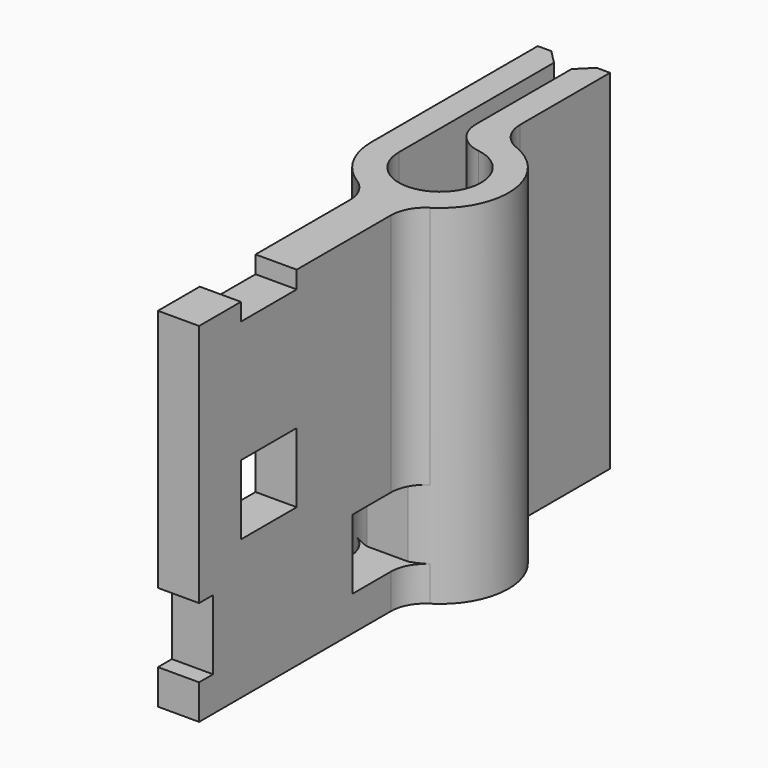
from build123d import *

# Parameters (mm, degrees)
F1_DEPTH = 25.4
F2_SIZE  = 1.016
F3_W     = 3
F3_H     = 19.05
F4_DEPTH = 25.4
F5_W     = 5.08
F5_H     = 5.08
F5_W_2   = 1.27
F5_H_2   = 1.27
F6_DEPTH = 6.501
F7_R     = 2.5


with BuildPart() as f1:
    # F0 (on Top) → F1 (new body)
    with BuildSketch(Plane.XY):
        with BuildLine():
            Line((0.635, 15.1509385957), (0.635, 2.4509385957))
            ThreePointArc((0.635, 2.4509385957), (5.0286441204, -1.3802173742), (-0.635, 0))
            Line((-0.635, 0), (-0.635, 15.1509385957))
            Line((-0.635, 15.1509385957), (-2.635, 15.1509385957))
            Line((-2.635, 15.1509385957), (-2.635, 0))
            ThreePointArc((-2.635, 0), (5.8037497728, -3.6297382826), (2.635, 4.9927046778))
            Line((2.635, 4.9927046778), (2.635, 15.1509385957))
            Line((2.635, 15.1509385957), (0.635, 15.1509385957))
        make_face()
    extrude(amount=F1_DEPTH)

    # F2
    f2_edges = [f1.edges().sort_by_distance(p)[0] for p in [
        (-0.635, 15.150939, 12.7),
        (0.635, 15.150939, 12.7),
    ]]
    chamfer(f2_edges, length=F2_SIZE)

    # F3 (on Top) → F4 (join, through all)
    with BuildSketch(Plane.XY):
        with Locations((2.365, -14.2946960071)):
            Rectangle(F3_W, F3_H)
    extrude(amount=F4_DEPTH)

    # F5 (on face) → F6 (cut, through all)
    with BuildSketch(Plane.YZ.offset(3.865)):
        with Locations((-7.3096960071, 5.08)):
            Rectangle(F5_W, F5_H)
        with Locations((-17.4696960071, 12.7)):
            Rectangle(F5_W, F5_H)
        with Locations((-23.1846960071, 5.08)):
            Rectangle(F5_W_2, F5_H)
        with Locations((-17.4696960071, 24.765)):
            Rectangle(F5_W, F5_H_2)
    extrude(amount=-F6_DEPTH, mode=Mode.SUBTRACT)

    # F7
    f7_edges = [f1.edges().sort_by_distance(p)[0] for p in [
        (0.635, 2.450939, 12.7),
        (-2.635, 0, 12.7),
        (2.635, 4.992705, 12.7),
        (3.865, -4.769696, 16.51),
        (0.865, -4.769696, 16.51),
        (0.865, -4.769696, 1.27),
        (3.865, -4.769696, 1.27),
    ]]
    fillet(f7_edges, radius=F7_R)


solid = f1.part
